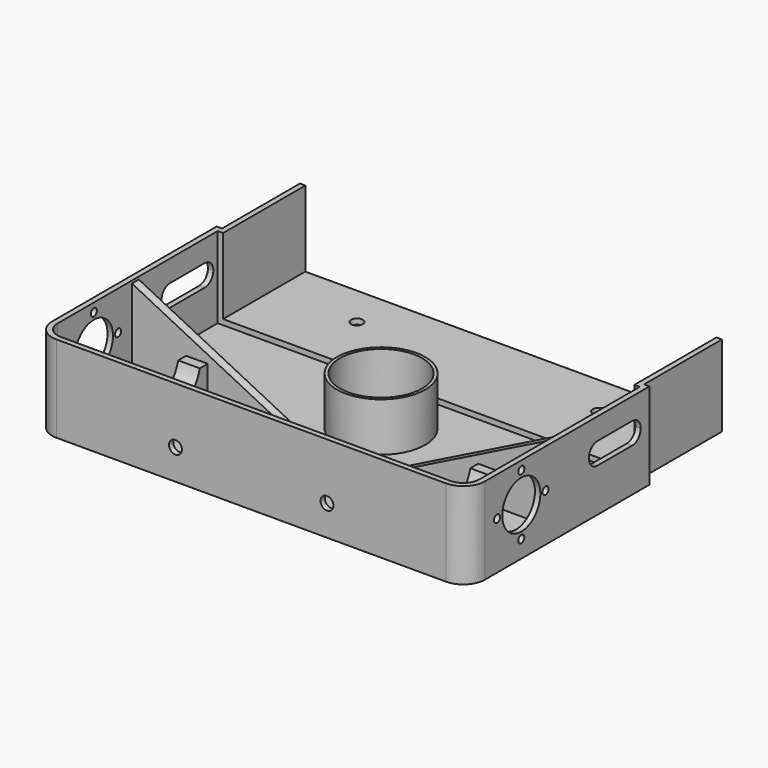
from build123d import *

# Parameters (mm, degrees)
F0_W             = 200
F0_H             = 150
F1_DEPTH         = 40
F2_R             = 10
F3_W             = 200
F3_H             = 100
F4_DEPTH         = 2.5
F5_W             = 40
F5_H             = 60
F6_DEPTH         = 200
F7_T             = 2.5
F7_T3_DEPTH      = 42.5
F7_T5_DEPTH      = 200
F9_DEPTH         = 150
F10_R            = 6
F11_DEPTH        = 25
F12_R            = 20.4
F12_R_2          = 19
F13_DEPTH        = 25
F14_R            = 2.75
F15_DEPTH        = 25
F16_R            = 3
F17_DEPTH        = 200
F18_R            = 1.75
F19_DEPTH        = 12.5
F19_COPIES_COUNT = 4
F21_START        = -28
F21_DEPTH        = 4
F22_R            = 3.5
F23_DEPTH        = 25
F24_W            = 10
F24_H            = 50.5
F25_DEPTH        = 15
F26_R            = 18
F26_R_2          = 1.75
F26_R_3          = 11
F27_DEPTH        = 95
F28_DEPTH        = 400
F28_DEPTH_BACK   = 100.001
F28_COPIES_COUNT = 4
F29_DEPTH        = 195


# Not quite as in the source:
# - a pattern or mirror of a feature is missing from the dataset's text; its kind, count and spacing are read off the source's solid
# - a shell that OpenCascade refuses in one call is made with other operations: the cavity is built on its own and cut out


with BuildPart() as f1:
    # F0 (on Top) → F1 (new body)
    with BuildSketch(Plane.XY):
        with Locations((0, 50)):
            Rectangle(F0_W, F0_H)
    extrude(amount=F1_DEPTH)

    # F2
    f2_edges = [f1.edges().sort_by_distance(p)[0] for p in [
        (-100, -25, 20),
        (100, -25, 20),
    ]]
    fillet(f2_edges, radius=F2_R)

    # F3 (on Top) → F4 (cut)
    with BuildSketch(Plane.XY):
        with Locations((0, 130)):
            Rectangle(F3_W, F3_H)
    extrude(amount=F4_DEPTH, mode=Mode.SUBTRACT)

    # F5 (on Top) → F6 (cut)
    with BuildSketch(Plane.XY):
        with Locations((-117.5, 110)):
            Rectangle(F5_W, F5_H)
        with Locations((117.5, 110)):
            Rectangle(F5_W, F5_H)
    extrude(amount=F6_DEPTH, mode=Mode.SUBTRACT)

    # F7: shell of thickness 2.5, made by hand


with BuildPart() as f7_core1:
    # F7_t2: copy of F1
    add(f1.part)

    # the walls: a layer under each face that stays
    f7_faces = [f7_core1.faces().sort_by_distance(p)[0] for p in [
        (-100, 32.5, 20),
        (-97.0710678119, -22.0710678119, 20),
        (0, -25, 20),
        (97.0710678119, -22.0710678119, 20),
        (100, 32.5, 20),
        (97.5, 102.5, 21.25),
        (0, 102.5, 2.5),
        (-97.5, 102.5, 21.25),
        (-93.3333333333, 80, 1.3333333333),
        (0, 27.5, 0),
    ]]
    thicken(f7_faces, amount=-F7_T, mode=Mode.SUBTRACT)

    # F7_s4 → F7_t3 (cut)
    with BuildSketch(Plane.XY):
        Polygon((97.525, 80.025), (95, 80), (95, 77.5), (97.5, 77.5), align=None)
        Polygon((-97.525, 80.025), (-95, 80), (-95, 77.5), (-97.5, 77.5), align=None)
    extrude(amount=F7_T3_DEPTH, mode=Mode.SUBTRACT)

    # F7_s6 → F7_t5 (cut)
    with BuildSketch(Plane.YZ.offset(-100)):
        Polygon((80.025, 2.475), (80, 5), (77.5, 5), (77.5, 2.5), align=None)
    extrude(amount=F7_T5_DEPTH, mode=Mode.SUBTRACT)


with BuildPart() as f1_1:
    add(f1.part)

    # what is left inside the walls is the cavity
    f7_cavity = [f7_core1.part.solids().sort_by_distance(p)[0] for p in [
        (0, 26.666667, 39.975),
    ]]
    add(f7_cavity, mode=Mode.SUBTRACT)

    # F8 (on Right) → F9 (cut, symmetric)
    with BuildSketch(Plane.YZ):
        with BuildLine():
            Line((50, 20), (50, 30))
            ThreePointArc((50, 30), (45, 25), (50, 20))
        make_face()
        with BuildLine():
            ThreePointArc((55, 25), (53.5355339059, 28.5355339059), (50, 30))
            Line((50, 30), (50, 20))
            ThreePointArc((50, 20), (53.5355339059, 21.4644660941), (55, 25))
        make_face()
        with BuildLine():
            Line((70, 30), (50, 30))
            ThreePointArc((50, 30), (53.5355339059, 28.5355339059), (55, 25))
            ThreePointArc((55, 25), (53.5355339059, 21.4644660941), (50, 20))
            Line((50, 20), (70, 20))
            ThreePointArc((70, 20), (65, 25), (70, 30))
        make_face()
        with BuildLine():
            Line((70, 20), (70, 30))
            ThreePointArc((70, 30), (65, 25), (70, 20))
        make_face()
        with BuildLine():
            ThreePointArc((75, 25), (73.5355339059, 28.5355339059), (70, 30))
            Line((70, 30), (70, 20))
            ThreePointArc((70, 20), (73.5355339059, 21.4644660941), (75, 25))
        make_face()
    extrude(amount=F9_DEPTH, both=True, mode=Mode.SUBTRACT)

    # F10 (on Top) → F11 (cut)
    with BuildSketch(Plane.XY):
        with Locations((0, 50)):
            Circle(F10_R)
    extrude(amount=F11_DEPTH, mode=Mode.SUBTRACT)

    # F12 (on Top) → F13 (join)
    with BuildSketch(Plane.XY):
        with Locations((0, 50)):
            Circle(F12_R)
        with Locations((0, 50)):
            Circle(F12_R_2, mode=Mode.SUBTRACT)
    extrude(amount=F13_DEPTH)

    # F14 (on Top) → F15 (cut)
    with BuildSketch(Plane.XY):
        with Locations((-55.8614357137, -5.8614357137)):
            Circle(F14_R)
        with Locations((55.8614357137, -5.8614357137)):
            Circle(F14_R)
        with Locations((55.8614357137, 105.8614357137)):
            Circle(F14_R)
        with BuildLine():
            ThreePointArc((-53.9168920655, 103.9168920655), (-53.3207669993, 104.8090562747), (-53.1114357137, 105.8614357137))
            ThreePointArc((-53.1114357137, 105.8614357137), (-58.4021044281, 106.9138151527), (-53.9168920655, 103.9168920655))
        make_face()
    extrude(amount=F15_DEPTH, mode=Mode.SUBTRACT)

    # F16 (on Front) → F17 (cut)
    with BuildSketch(Plane.XZ):
        with Locations((-35, 14)):
            Circle(F16_R)
        with Locations((35, 14)):
            Circle(F16_R)
    extrude(amount=F17_DEPTH, mode=Mode.SUBTRACT)

    # F18 (on Top) → F19 (cut, symmetric)
    with BuildSketch(Plane.XY):
        with Locations((0, 39)):
            Circle(F18_R)
    f19 = extrude(amount=F19_DEPTH, both=True, mode=Mode.SUBTRACT)

    # F19_copies: F19 ×4 about axis
    f19_copies_axis = Axis((0, 50, 0), (0, 0, 1))
    for i in range(1, F19_COPIES_COUNT):
        add(f19.rotate(f19_copies_axis, i * 360 / F19_COPIES_COUNT), mode=Mode.SUBTRACT)

    # F20 (on Front) → F21 (join)
    with BuildSketch(Plane.XZ.offset(F21_START)):
        Polygon((-100, 40), (-100, 0), (-20, 0), align=None)
        Polygon((100, 40), (20, 0), (100, 0), align=None)
    extrude(amount=-F21_DEPTH)

    # F22 (on Top) → F23 (cut)
    with BuildSketch(Plane.XY):
        with Locations((0, -15)):
            Circle(F22_R)
    extrude(amount=F23_DEPTH, mode=Mode.SUBTRACT)

    # F24 (on face) → F25 (join)
    with BuildSketch(Plane.XY.offset(2.5)):
        with Locations((-67.5, 2.75)):
            Rectangle(F24_W, F24_H)
        with Locations((67.5, 2.75)):
            Rectangle(F24_W, F24_H)
    extrude(amount=F25_DEPTH)

    # F26 (on Right) → F27 (cut, symmetric)
    with BuildSketch(Plane.YZ):
        with Locations((6, 22)):
            Circle(F26_R)
        with Locations((-8, 22)):
            Circle(F26_R_2, mode=Mode.SUBTRACT)
        with Locations((6, 22)):
            Circle(F26_R_3, mode=Mode.SUBTRACT)
    extrude(amount=F27_DEPTH, both=True, mode=Mode.SUBTRACT)

    # F26 (on Right) → F28 (cut, two sides)
    with BuildSketch(Plane.YZ) as f28_sk:
        with Locations((-8, 22)):
            Circle(F26_R_2)
    f28 = extrude(amount=-F28_DEPTH, mode=Mode.SUBTRACT) + extrude(f28_sk.sketch, amount=F28_DEPTH_BACK, mode=Mode.SUBTRACT)

    # F28_copies: F28 ×4 about axis
    f28_copies_axis = Axis((0, 6, 22), (1, 0, 0))
    for i in range(1, F28_COPIES_COUNT):
        add(f28.rotate(f28_copies_axis, i * 360 / F28_COPIES_COUNT), mode=Mode.SUBTRACT)

    # F26 (on Right) → F29 (cut, symmetric)
    with BuildSketch(Plane.YZ):
        with Locations((6, 22)):
            Circle(F26_R_3)
    extrude(amount=F29_DEPTH, both=True, mode=Mode.SUBTRACT)


solid = f1_1.part
